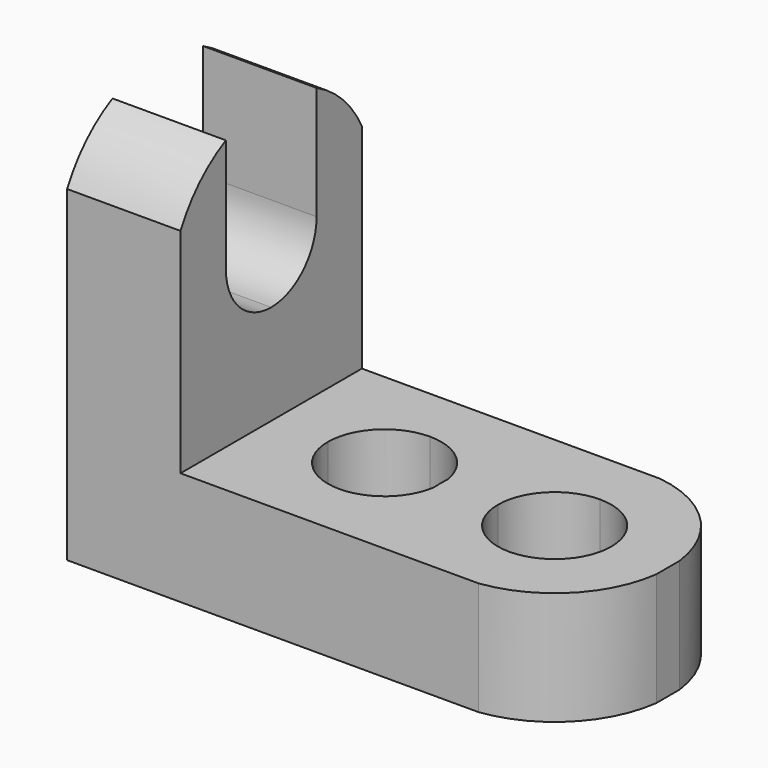
from build123d import *

# Parameters (mm, degrees)
F0_W     = 57.15
F0_H     = 44.45
F1_DEPTH = 25.4
F2_W     = 44.45
F2_H     = 31.75
F3_DEPTH = 25.4
F5_DEPTH = 25.4
F7_DEPTH = 25.4


with BuildPart() as f1:
    # F0 (on Front) → F1 (new body)
    with BuildSketch(Plane.XZ):
        with Locations((28.575, 22.225)):
            Rectangle(F0_W, F0_H)
    extrude(amount=F1_DEPTH)

    # F2 (on face) → F3 (cut)
    with BuildSketch(Plane.XZ.offset(25.4)):
        with Locations((34.925, 28.575)):
            Rectangle(F2_W, F2_H)
    extrude(amount=-F3_DEPTH, mode=Mode.SUBTRACT)

    # F4 (on face) → F5 (cut)
    with BuildSketch(Plane.YZ.offset(12.7)):
        with BuildLine():
            ThreePointArc((-19.05, 42.9509683429), (-15.9622689922, 44.0701615546), (-12.7, 44.45))
            Line((-12.7, 44.45), (-25.4, 44.45))
            Line((-25.4, 44.45), (-25.4, 36.6009683429))
            ThreePointArc((-25.4, 36.6009683429), (-22.740231571, 40.2911999139), (-19.05, 42.9509683429))
        make_face()
        with BuildLine():
            Line((0, 44.45), (-12.7, 44.45))
            ThreePointArc((-12.7, 44.45), (-9.4377310078, 44.0701615546), (-6.35, 42.9509683429))
            ThreePointArc((-6.35, 42.9509683429), (-2.659768429, 40.2911999139), (0, 36.6009683429))
            Line((0, 36.6009683429), (0, 44.45))
        make_face()
        with BuildLine():
            Line((-12.7, 36.6009683429), (-12.7, 44.45))
            ThreePointArc((-12.7, 44.45), (-15.9622689922, 44.0701615546), (-19.05, 42.9509683429))
            Line((-19.05, 42.9509683429), (-19.05, 30.2509683429))
            ThreePointArc((-19.05, 30.2509683429), (-17.1901280605, 34.7410964034), (-12.7, 36.6009683429))
        make_face()
        with BuildLine():
            ThreePointArc((-6.35, 42.9509683429), (-9.4377310078, 44.0701615546), (-12.7, 44.45))
            Line((-12.7, 44.45), (-12.7, 36.6009683429))
            ThreePointArc((-12.7, 36.6009683429), (-8.2098719395, 34.7410964034), (-6.35, 30.2509683429))
            Line((-6.35, 30.2509683429), (-6.35, 42.9509683429))
        make_face()
        with BuildLine():
            Line((-12.7, 23.9009683429), (-12.7, 30.2509683429))
            Line((-12.7, 30.2509683429), (-19.05, 30.2509683429))
            ThreePointArc((-19.05, 30.2509683429), (-17.1901280605, 25.7608402823), (-12.7, 23.9009683429))
        make_face()
        with BuildLine():
            Line((-12.7, 30.2509683429), (-12.7, 36.6009683429))
            ThreePointArc((-12.7, 36.6009683429), (-17.1901280605, 34.7410964034), (-19.05, 30.2509683429))
            Line((-19.05, 30.2509683429), (-12.7, 30.2509683429))
        make_face()
        with BuildLine():
            Line((-6.35, 30.2509683429), (-12.7, 30.2509683429))
            Line((-12.7, 30.2509683429), (-12.7, 23.9009683429))
            ThreePointArc((-12.7, 23.9009683429), (-8.2098719395, 25.7608402823), (-6.35, 30.2509683429))
        make_face()
        with BuildLine():
            ThreePointArc((-6.35, 30.2509683429), (-8.2098719395, 34.7410964034), (-12.7, 36.6009683429))
            Line((-12.7, 36.6009683429), (-12.7, 30.2509683429))
            Line((-12.7, 30.2509683429), (-6.35, 30.2509683429))
        make_face()
    extrude(amount=-F5_DEPTH, mode=Mode.SUBTRACT)

    # F6 (on face) → F7 (cut)
    with BuildSketch(Plane.XY.offset(12.7)):
        with BuildLine():
            ThreePointArc((31.6799919585, -11.7596803731), (29.5443618549, -7.8888915191), (25.4, -6.35))
            Line((25.4, -6.35), (25.4, -12.7))
            Line((25.4, -12.7), (31.6454185395, -12.7))
            ThreePointArc((31.6454185395, -12.7), (31.6540648134, -12.2295224974), (31.6799919585, -11.7596803731))
        make_face()
        with BuildLine():
            Line((25.4, -12.7), (25.4, -6.35))
            ThreePointArc((25.4, -6.35), (20.9098719395, -8.2098719395), (19.05, -12.7))
            Line((19.05, -12.7), (25.4, -12.7))
        make_face()
        with BuildLine():
            ThreePointArc((46.0831890214, 0), (44.45, 0.1045814605), (42.8168109786, 0))
            Line((42.8168109786, 0), (44.45, 0))
            Line((44.45, 0), (46.0831890214, 0))
        make_face()
        with BuildLine():
            Line((31.6454185395, -12.7), (25.4, -12.7))
            Line((25.4, -12.7), (25.4, -19.05))
            ThreePointArc((25.4, -19.05), (29.5443618549, -17.5111084809), (31.6799919585, -13.6403196269))
            ThreePointArc((31.6799919585, -13.6403196269), (31.6540648134, -13.1704775026), (31.6454185395, -12.7))
        make_face()
        with BuildLine():
            Line((25.4, -19.05), (25.4, -12.7))
            Line((25.4, -12.7), (19.05, -12.7))
            ThreePointArc((19.05, -12.7), (20.9098719395, -17.1901280605), (25.4, -19.05))
        make_face()
        with BuildLine():
            Line((57.15, 0), (46.0831890214, 0))
            ThreePointArc((46.0831890214, 0), (53.504206381, -3.645793619), (57.15, -11.0668109786))
            Line((57.15, -11.0668109786), (57.15, 0))
        make_face()
        with BuildLine():
            ThreePointArc((50.8, -12.7), (48.9401280605, -8.2098719395), (44.45, -6.35))
            Line((44.45, -6.35), (44.45, -12.7))
            Line((44.45, -12.7), (50.8, -12.7))
        make_face()
        with BuildLine():
            Line((44.45, -12.7), (44.45, -6.35))
            ThreePointArc((44.45, -6.35), (39.9598719395, -8.2098719395), (38.1, -12.7))
            Line((38.1, -12.7), (44.45, -12.7))
        make_face()
        with BuildLine():
            Line((44.45, -12.7), (38.1, -12.7))
            ThreePointArc((38.1, -12.7), (39.9598719395, -17.1901280605), (44.45, -19.05))
            Line((44.45, -19.05), (44.45, -12.7))
        make_face()
        with BuildLine():
            Line((50.8, -12.7), (44.45, -12.7))
            Line((44.45, -12.7), (44.45, -19.05))
            ThreePointArc((44.45, -19.05), (48.9401280605, -17.1901280605), (50.8, -12.7))
        make_face()
        with BuildLine():
            Line((57.15, -25.4), (57.15, -14.3331890214))
            ThreePointArc((57.15, -14.3331890214), (53.504206381, -21.754206381), (46.0831890214, -25.4))
            Line((46.0831890214, -25.4), (57.15, -25.4))
        make_face()
    extrude(amount=-F7_DEPTH, mode=Mode.SUBTRACT)


solid = f1.part
